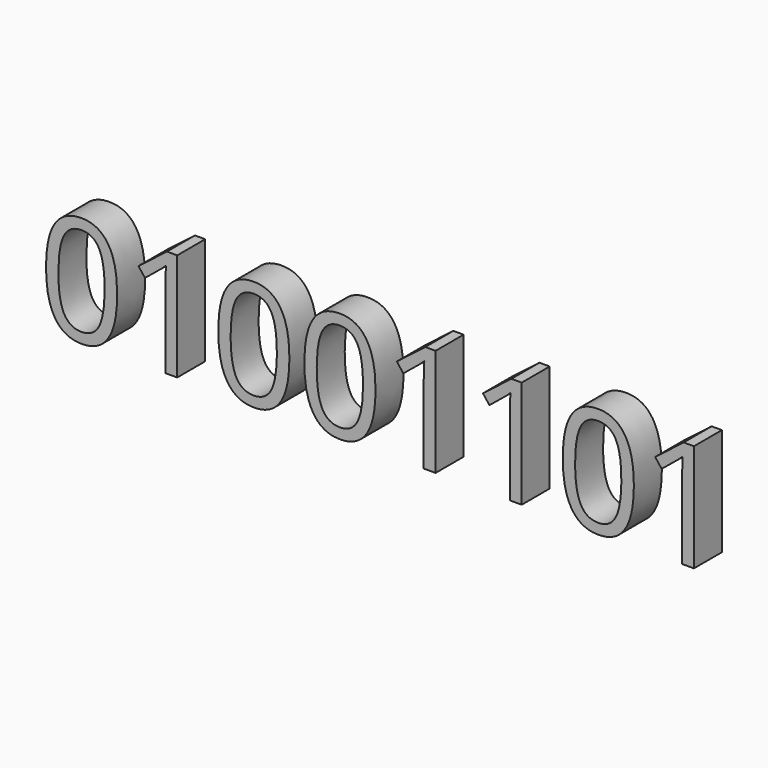
from build123d import *

# Parameters (mm, degrees)
F0_TEXT_SIZE = 109.3755217476
F1_DEPTH     = 25.4


# Not quite as in the source:
# - Text() gives the source's letters only with a copy of the font that has no kerning and outlines rounded to 1/6400 em; it was checked with that copy


with BuildPart() as f1:
    # F0 (on Front) → F1 (new body)
    with BuildSketch(Plane.XZ):
        with Locations((-33.0001041293, -34.1708064079)):
            Text('01001101', F0_TEXT_SIZE, font='Open Sans', text_align=(TextAlign.LEFT, TextAlign.BOTTOM))
    extrude(amount=F1_DEPTH)


solid = f1.part
